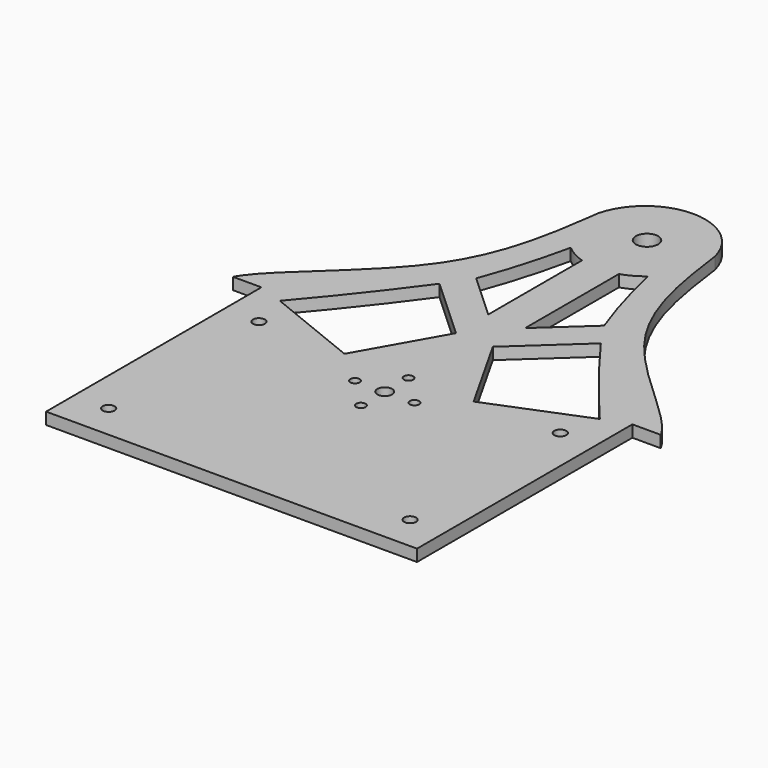
from build123d import *

# Parameters (mm, degrees)
F0_R     = 1.6
F0_R_2   = 1.25
F0_R_3   = 2
F0_R_4   = 3
F1_DEPTH = 3.175


# Not quite as in the source:
# - a feature names something its author has since deleted; it is built from what else it names


with BuildPart() as f1:
    # F0 (on Top) → F1 (new body)
    with BuildSketch(Plane.XY):
        with BuildLine():
            Line((-49.8799999985, 8.89), (-49.8799999985, -63.5))
            Line((-49.8799999985, -63.5), (49.8799999985, -63.5))
            Line((49.8799999985, -63.5), (49.8799999985, 8.89))
            Line((49.8799999985, 8.89), (57.4999999985, 8.89))
            add(Edge.make_bspline(
                [(15.7093216459, 79.3836478465), (17.5511050126, 65.7915878149), (21.2374579051, 38.4486252292), (53.8863670451, 16.0459412112), (57.4999999985, 8.89)],
                knots=[0, 0, 0, 0, 0.4099092451, 0.8244764195, 0.8244764195, 0.8244764195, 0.8244764195], degree=3))
            ThreePointArc((15.7093216459, 79.3836478465), (0, 91.6600956823), (-15.7093216459, 79.3836478465))
            add(Edge.make_bspline(
                [(-15.7093216459, 79.3836478465), (-15.8351413169, 78.4551192516), (-15.960918893, 77.5265804672), (-16.0889396188, 76.5984215036)],
                knots=[0, 0, 0, 0, 0.0280025584, 0.0280025584, 0.0280025584, 0.0280025584], degree=3))
            add(Edge.make_bspline(
                [(-16.0889396188, 76.5984215036), (-17.8349219122, 63.9399312026), (-22.3463470917, 37.6877393462), (-53.8863670451, 16.0459412112), (-57.4999999985, 8.89)],
                knots=[0.0280025584, 0.0280025584, 0.0280025584, 0.0280025584, 0.4099092451, 0.8244764195, 0.8244764195, 0.8244764195, 0.8244764195], degree=3))
            Line((-57.4999999985, 8.89), (-49.8799999985, 8.89))
        make_face()
        with Locations((-40.5299999985, -54.15)):
            Circle(F0_R, mode=Mode.SUBTRACT)
        with Locations((-40.5299999985, -3.635)):
            Circle(F0_R, mode=Mode.SUBTRACT)
        with Locations((-8, -12)):
            Circle(F0_R_2, mode=Mode.SUBTRACT)
        with Locations((40.5299999985, -54.15)):
            Circle(F0_R, mode=Mode.SUBTRACT)
        with Locations((0, -20)):
            Circle(F0_R_2, mode=Mode.SUBTRACT)
        with Locations((0, -12)):
            Circle(F0_R_3, mode=Mode.SUBTRACT)
        with Locations((8, -12)):
            Circle(F0_R_2, mode=Mode.SUBTRACT)
        with Locations((0, -4)):
            Circle(F0_R_2, mode=Mode.SUBTRACT)
        with Locations((40.5299999985, -3.635)):
            Circle(F0_R, mode=Mode.SUBTRACT)
        with BuildLine():
            Line((-21.7048343448, 33.51030308), (-4.9567933963, 18.14211905))
            Line((-4.9567933963, 18.14211905), (-17.3775311559, -3.8353991695))
            Line((-17.3775311559, -3.8353991695), (-43.0274941027, 6.520065479))
            ThreePointArc((-43.0274941027, 6.520065479), (-32.1093228463, 19.8122760508), (-21.7048343448, 33.51030308))
        make_face(mode=Mode.SUBTRACT)
        with BuildLine():
            ThreePointArc((-10.4206144746, 63.5413418448), (-7.8378238948, 61.7519957694), (-4.9567933963, 60.4981098798))
            Line((-4.9567933963, 60.4981098798), (-4.9567933963, 29.0021225758))
            Line((-4.9567933963, 29.0021225758), (-17.2076895833, 40.2436777949))
            ThreePointArc((-17.2076895833, 40.2436777949), (-13.397490451, 51.7711279758), (-10.4206144746, 63.5413418448))
        make_face(mode=Mode.SUBTRACT)
        with Locations((-0.0292583045, 76.2)):
            Circle(F0_R_4, mode=Mode.SUBTRACT)
        with BuildLine():
            Line((17.3775311559, -3.8353991695), (4.9567933963, 18.14211905))
            Line((4.9567933963, 18.14211905), (21.7048343448, 33.51030308))
            ThreePointArc((21.7048343448, 33.51030308), (32.1093228463, 19.8122760508), (43.0274941027, 6.520065479))
            Line((43.0274941027, 6.520065479), (17.3775311559, -3.8353991695))
        make_face(mode=Mode.SUBTRACT)
        with BuildLine():
            Line((17.2076895833, 40.2436777949), (4.9567933963, 29.0021225758))
            Line((4.9567933963, 29.0021225758), (4.9567933963, 60.4981098798))
            ThreePointArc((4.9567933963, 60.4981098798), (7.8378238948, 61.7519957694), (10.4206144746, 63.5413418448))
            ThreePointArc((10.4206144746, 63.5413418448), (13.397490451, 51.7711279758), (17.2076895833, 40.2436777949))
        make_face(mode=Mode.SUBTRACT)
    extrude(amount=F1_DEPTH)


solid = f1.part
